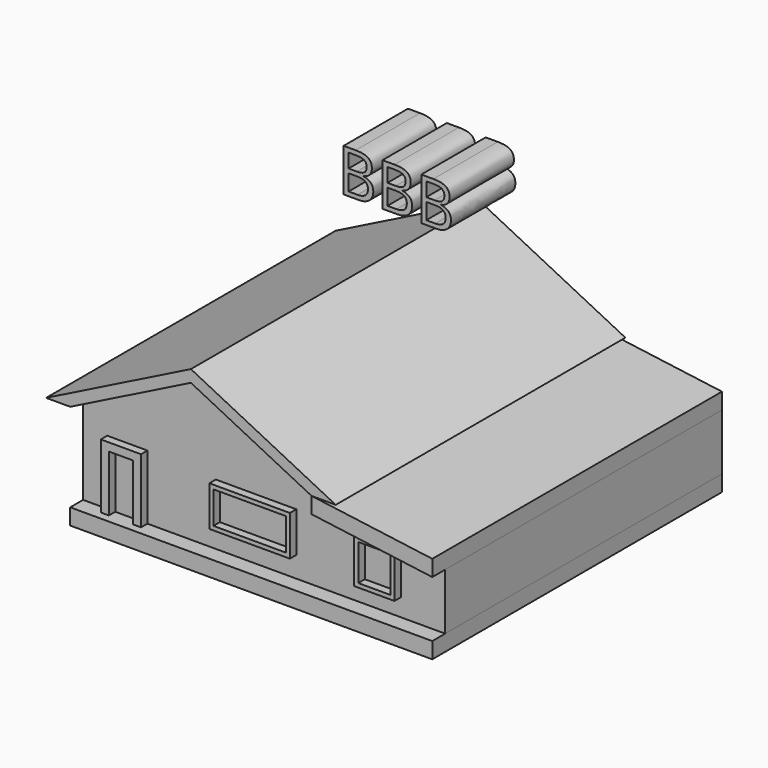
from build123d import *

# Parameters (mm, degrees)
F1_DEPTH     = 13716
F0_W         = 4572
F0_H         = 609.6
F0_W_2       = 3048
F0_H_2       = 1524
F0_W_3       = 1524
F0_H_3       = 1676.4
F2_DEPTH     = 13106.4
F0_W_4       = 914.4
F0_H_4       = 2133.6
F0_W_5       = 2743.2
F0_H_5       = 1219.2
F0_W_6       = 1209.2
F0_H_6       = 1361.6
F3_DEPTH     = 13411.2
F0_W_7       = 1219.2
F0_H_7       = 1371.6
F4_W         = 3520.1352
F4_H         = 1837.6392
F4_W_2       = 3215.3352
F4_H_2       = 1532.8392
F5_DEPTH     = 304.8
F0_TEXT_SIZE = 2271.7247406642
F6_DEPTH     = 3048


# Not quite as in the source:
# - Text() gives the source's letters only with a copy of the font that has no kerning and outlines rounded to 1/6400 em; it was checked with that copy


with BuildPart() as f1:
    # F0 (on Front) → F1 (new body)
    with BuildSketch(Plane.XZ):
        Polygon((0, 2286), (4572, 0), (5486.4, 0), (0, 2743.2), align=None)
        Polygon((-5486.4, 0), (-4572, 0), (0, 2286), (0, 2743.2), align=None)
    extrude(amount=F1_DEPTH)


with BuildPart() as f1b:
    # F0 (on Front) → F1, piece 2 (new body)
    with BuildSketch(Plane.XZ):
        Polygon((9144, -609.6), (4572, 0), (4572, -609.6), (9144, -1219.2), align=None)
    extrude(amount=F1_DEPTH)


with BuildPart() as f1c:
    # F0 (on Front) → F1, piece 3 (new body)
    with BuildSketch(Plane.XZ):
        with Locations((6858, -3657.6)):
            Rectangle(F0_W, F0_H)
        Polygon((-3657.6, -3352.8), (-4572, -3352.8), (-4572, -3962.4), (4572, -3962.4), (4572, -3352.8), (-2133.6, -3352.8), (-2438.4, -3352.8), (-3352.8, -3352.8), align=None)
    extrude(amount=F1_DEPTH)


with BuildPart() as f2:
    # F0 (on Front) → F2 (new body)
    with BuildSketch(Plane.XZ):
        Polygon((4572, 0), (0, 0), (-4572, 0), (-4572, -3352.8), (-3657.6, -3352.8), (-3657.6, -914.4), (-2133.6, -914.4), (-2133.6, -3352.8), (4572, -3352.8), (4572, -609.6), align=None)
        with Locations((1981.2, -1800.8599634171)):
            Rectangle(F0_W_2, F0_H_2, mode=Mode.SUBTRACT)
        Polygon((9144, -1219.2), (4572, -609.6), (4572, -3352.8), (9144, -3352.8), align=None)
        with Locations((6705.6, -1847.3336965561)):
            Rectangle(F0_W_3, F0_H_3, mode=Mode.SUBTRACT)
        Polygon((-4572, 0), (0, 0), (4572, 0), (0, 2286), align=None)
    extrude(amount=F2_DEPTH)

    # F4 (on face) → F5 (join)
    with BuildSketch(Plane(origin=(-4572, 0, 0), x_dir=(0, -1, 0), z_dir=(-1, 0, 0))):
        with Locations((2977.7692902924, -1433.9702620605)):
            Rectangle(F4_W, F4_H)
        with Locations((2977.7692902924, -1433.9702620605)):
            Rectangle(F4_W_2, F4_H_2, mode=Mode.SUBTRACT)
        with Locations((10128.6564, -1433.9316)):
            Rectangle(F4_W, F4_H)
        with Locations((10128.6564, -1433.9316)):
            Rectangle(F4_W_2, F4_H_2, mode=Mode.SUBTRACT)
    extrude(amount=F5_DEPTH)


with BuildPart() as f2b:
    # F0 (on Front) → F2, piece 2 (new body)
    with BuildSketch(Plane.XZ):
        with Locations((-2895.6, -2286)):
            Rectangle(F0_W_4, F0_H_4)
    extrude(amount=F2_DEPTH)


with BuildPart() as f2c:
    # F0 (on Front) → F2, piece 3 (new body)
    with BuildSketch(Plane.XZ):
        with Locations((1981.2, -1800.8599634171)):
            Rectangle(F0_W_5, F0_H_5)
    extrude(amount=F2_DEPTH)


with BuildPart() as f2d:
    # F0 (on Front) → F2, piece 4 (new body)
    with BuildSketch(Plane.XZ):
        with Locations((6705.6, -1847.3336965561)):
            Rectangle(F0_W_6, F0_H_6)
    extrude(amount=F2_DEPTH)


with BuildPart() as f3:
    # F0 (on Front) → F3 (new body)
    with BuildSketch(Plane.XZ):
        Polygon((-3657.6, -914.4), (-3657.6, -3352.8), (-3352.8, -3352.8), (-3352.8, -1219.2), (-2438.4, -1219.2), (-2438.4, -3352.8), (-2133.6, -3352.8), (-2133.6, -914.4), align=None)
    extrude(amount=F3_DEPTH)


with BuildPart() as f3b:
    # F0 (on Front) → F3, piece 2 (new body)
    with BuildSketch(Plane.XZ):
        with Locations((1981.2, -1800.8599634171)):
            Rectangle(F0_W_2, F0_H_2)
        with Locations((1981.2, -1800.8599634171)):
            Rectangle(F0_W_5, F0_H_5, mode=Mode.SUBTRACT)
    extrude(amount=F3_DEPTH)


with BuildPart() as f3c:
    # F0 (on Front) → F3, piece 3 (new body)
    with BuildSketch(Plane.XZ):
        with Locations((6705.6, -1847.3336965561)):
            Rectangle(F0_W_3, F0_H_3)
        with Locations((6705.6, -1847.3336965561)):
            Rectangle(F0_W_7, F0_H_7, mode=Mode.SUBTRACT)
    extrude(amount=F3_DEPTH)


with BuildPart() as f6:
    # F0 (on Front) → F6 (new body)
    with BuildSketch(Plane.XZ):
        with Locations((-2972.1286296844, 3337.4259471893)):
            Text('BBB', F0_TEXT_SIZE, font='Open Sans', text_align=(TextAlign.LEFT, TextAlign.BOTTOM))
    extrude(amount=F6_DEPTH)


solid = Compound([f1.part, f1b.part, f1c.part, f2.part, f2b.part, f2c.part, f2d.part, f3.part, f3b.part, f3c.part, f6.part])
